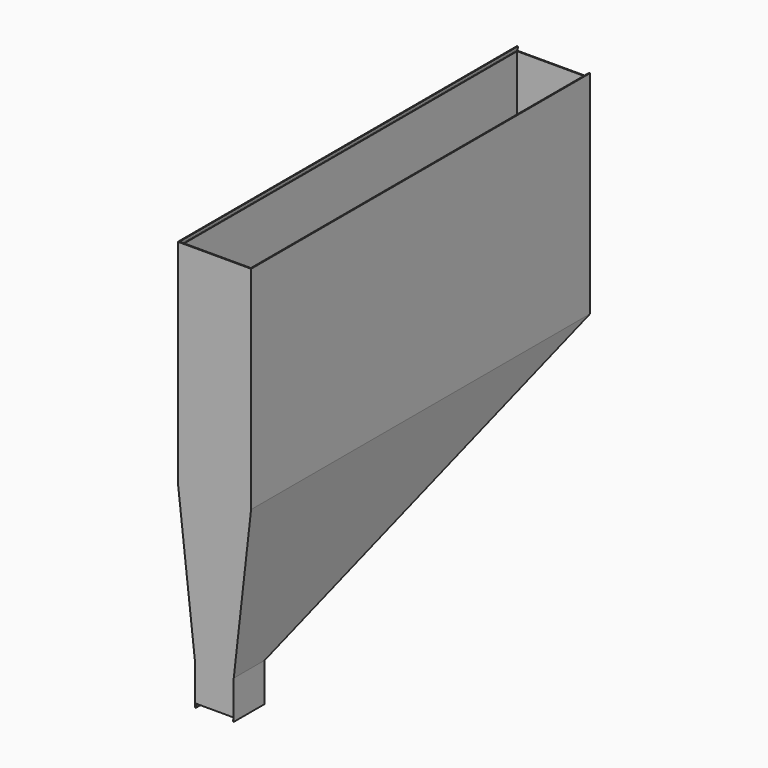
from build123d import *

# Parameters (mm, degrees)
F0_W        = 100
F0_H        = 100
F0_W_2      = 190
F0_H_2      = 550
F1_DEPTH    = 550
F3_DEPTH    = 190
F4_T        = 2.5
F4_T3_DEPTH = 105
F4_T5_DEPTH = 105
F6_DEPTH    = 98.5
F7_W        = 185
F7_H        = 5
F8_DEPTH    = 2.5
F9_DEPTH    = 1099


# Not quite as in the source:
# - a shell that OpenCascade refuses in one call is made with other operations: the cavity is built on its own and cut out


with BuildPart() as f1:
    # F0 (on Front) → F1 (new body, symmetric)
    with BuildSketch(Plane.XZ):
        with Locations((0, -450)):
            Rectangle(F0_W, F0_H)
        with Locations((0, 275)):
            Rectangle(F0_W_2, F0_H_2)
        Polygon((50, -400), (95, 0), (-95, 0), (-50, -400), align=None)
    extrude(amount=F1_DEPTH, both=True)

    # F2 (on face) → F3 (cut)
    with BuildSketch(Plane.YZ.offset(95)):
        Polygon((550, -500), (550, 0), (-450, -400), (-450, -500), align=None)
    extrude(amount=-F3_DEPTH, mode=Mode.SUBTRACT)

    # F4: shell of thickness 2.5, made by hand


with BuildPart() as f4_core1:
    # F4_t2: copy of F1
    add(f1.part)

    # the walls: a layer under each face that stays
    f4_faces = [f4_core1.faces().sort_by_distance(p)[0] for p in [
        (50, -500, -450),
        (0, -550, 25),
        (72.5, 0, -200),
        (0, -450, -450),
        (-50, -500, -450),
        (95, 0, 275),
        (-95, 0, 275),
        (-72.5, 0, -200),
        (0, 50, -200),
        (0, 550, 275),
    ]]
    thicken(f4_faces, amount=-F4_T, mode=Mode.SUBTRACT)

    # F4_s4 → F4_t3 (cut)
    with BuildSketch(Plane.XZ.offset(447.5)):
        Polygon((50.0498432829, -400.0027948693), (47.5, -400), (47.5, -399.8598171527), (47.5156717096, -399.7205130673), align=None)
        Polygon((-50.0498432829, -400.0027948693), (-47.5, -400), (-47.5, -399.8598171527), (-47.5156717096, -399.7205130673), align=None)
    extrude(amount=F4_T3_DEPTH, mode=Mode.SUBTRACT)

    # F4_s6 → F4_t5 (cut)
    with BuildSketch(Plane.YZ.offset(-52.5)):
        Polygon((-449.9657152331, -400.0232119173), (-452.5, -400), (-452.5, -398.3074175964), (-450.9284766909, -397.6788082728), align=None)
    extrude(amount=F4_T5_DEPTH, mode=Mode.SUBTRACT)


with BuildPart() as f1_1:
    add(f1.part)

    # what is left inside the walls is the cavity
    f4_cavity = [f4_core1.part.solids().sort_by_distance(p)[0] for p in [
        (-92.475, 182.5, 275.070091),
    ]]
    add(f4_cavity, mode=Mode.SUBTRACT)

    # F5 (on face) → F6 (cut)
    with BuildSketch(Plane.XZ.offset(550)):
        Polygon((-48.5, -495), (-48.5, -500), (48.5, -500), (48.5, -495), (49.5, -495), (49.5, -490), (-49.5, -490), (-49.5, -495), align=None)
    extrude(amount=-F6_DEPTH, mode=Mode.SUBTRACT)

    # F7 (on face) → F8 (cut)
    with BuildSketch(Plane(origin=(0, 550, 0), x_dir=(-1, 0, 0), z_dir=(0, 1, 0))):
        with Locations((0, 547.5)):
            Rectangle(F7_W, F7_H)
    extrude(amount=-F8_DEPTH, mode=Mode.SUBTRACT)

    # F7 (on face) → F9 (cut)
    with BuildSketch(Plane(origin=(0, 550, 0), x_dir=(-1, 0, 0), z_dir=(0, 1, 0))):
        Polygon((92.5, 545), (-92.5, 545), (-94, 545), (-94, 540), (94, 540), (94, 545), align=None)
    extrude(amount=-F9_DEPTH, mode=Mode.SUBTRACT)


solid = f1_1.part
